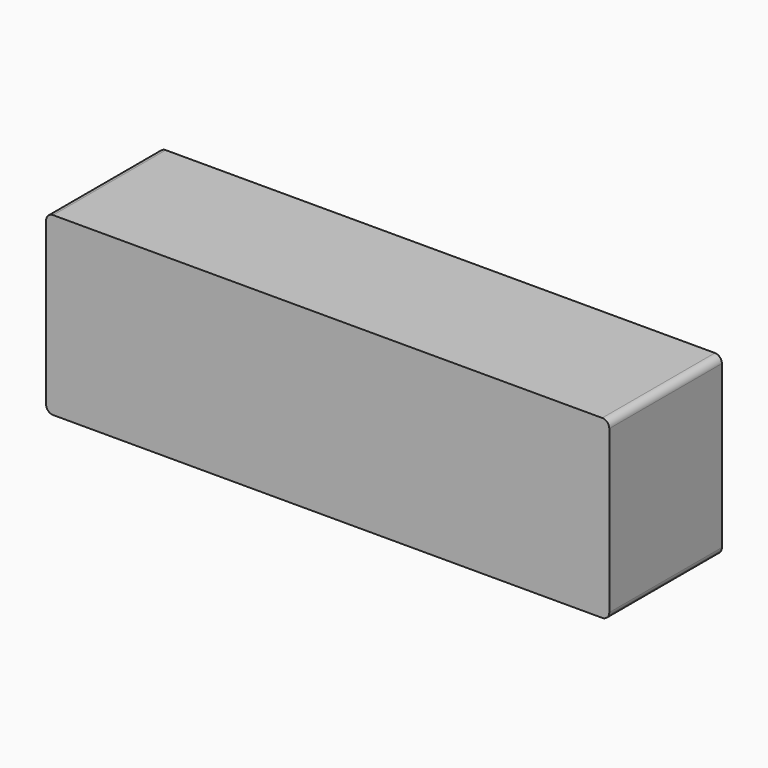
from build123d import *

# Parameters (mm, degrees)
F0_W     = 6.35
F0_H     = 6.35
F1_DEPTH = 25.4
F2_R     = 1.27


with BuildPart() as f1:
    # F0 (on Front) → F1 (new body)
    with BuildSketch(Plane.XZ):
        Polygon((-50.8, 15.875), (-50.8, 9.525), (-44.45, 9.525), (-38.1, 9.525), (-38.1, 15.875), align=None)
        with Locations((-47.625, 6.35)):
            Rectangle(F0_W, F0_H)
        Polygon((-50.8, 3.175), (-50.8, -3.175), (-44.45, -3.175), (-38.1, -3.175), (-38.1, 3.175), (-44.45, 3.175), align=None)
        with Locations((-47.625, -6.35)):
            Rectangle(F0_W, F0_H)
        Polygon((-50.8, -15.875), (0, -15.875), (0, -9.525), (-6.35, -9.525), (-44.45, -9.525), (-50.8, -9.525), align=None)
        Polygon((0, -15.875), (50.8, -15.875), (50.8, -9.525), (44.45, -9.525), (6.35, -9.525), (0, -9.525), align=None)
        with Locations((3.175, -6.35)):
            Rectangle(F0_W, F0_H)
        with Locations((-3.175, -6.35)):
            Rectangle(F0_W, F0_H)
        Polygon((-6.35, -3.175), (0, -3.175), (0, 3.175), (-6.35, 3.175), (-12.7, 3.175), (-12.7, -3.175), align=None)
        Polygon((0, 3.175), (0, -3.175), (6.35, -3.175), (12.7, -3.175), (12.7, 3.175), (6.35, 3.175), align=None)
        with Locations((3.175, 6.35)):
            Rectangle(F0_W, F0_H)
        with Locations((-3.175, 6.35)):
            Rectangle(F0_W, F0_H)
        Polygon((-6.35, 9.525), (0, 9.525), (0, 15.875), (-12.7, 15.875), (-12.7, 9.525), align=None)
        Polygon((0, 15.875), (0, 9.525), (6.35, 9.525), (12.7, 9.525), (12.7, 15.875), align=None)
        Polygon((44.45, 9.525), (50.8, 9.525), (50.8, 15.875), (38.1, 15.875), (38.1, 9.525), align=None)
        with Locations((47.625, 6.35)):
            Rectangle(F0_W, F0_H)
        Polygon((44.45, -3.175), (50.8, -3.175), (50.8, 3.175), (44.45, 3.175), (38.1, 3.175), (38.1, -3.175), align=None)
        with Locations((47.625, -6.35)):
            Rectangle(F0_W, F0_H)
        Polygon((-44.45, -9.525), (-6.35, -9.525), (-6.35, -3.175), (-12.7, -3.175), (-12.7, 3.175), (-6.35, 3.175), (-6.35, 9.525), (-12.7, 9.525), (-12.7, 15.875), (-38.1, 15.875), (-38.1, 9.525), (-44.45, 9.525), (-44.45, 3.175), (-38.1, 3.175), (-38.1, -3.175), (-44.45, -3.175), align=None)
        Polygon((6.35, -9.525), (44.45, -9.525), (44.45, -3.175), (38.1, -3.175), (38.1, 3.175), (44.45, 3.175), (44.45, 9.525), (38.1, 9.525), (38.1, 15.875), (12.7, 15.875), (12.7, 9.525), (6.35, 9.525), (6.35, 3.175), (12.7, 3.175), (12.7, -3.175), (6.35, -3.175), align=None)
    extrude(amount=F1_DEPTH)

    # F2
    f2_edges = [f1.edges().sort_by_distance(p)[0] for p in [
        (-50.8, -12.7, 15.875),
        (-50.8, -12.7, -15.875),
        (50.8, -12.7, 15.875),
        (50.8, -12.7, -15.875),
    ]]
    fillet(f2_edges, radius=F2_R)


solid = f1.part
